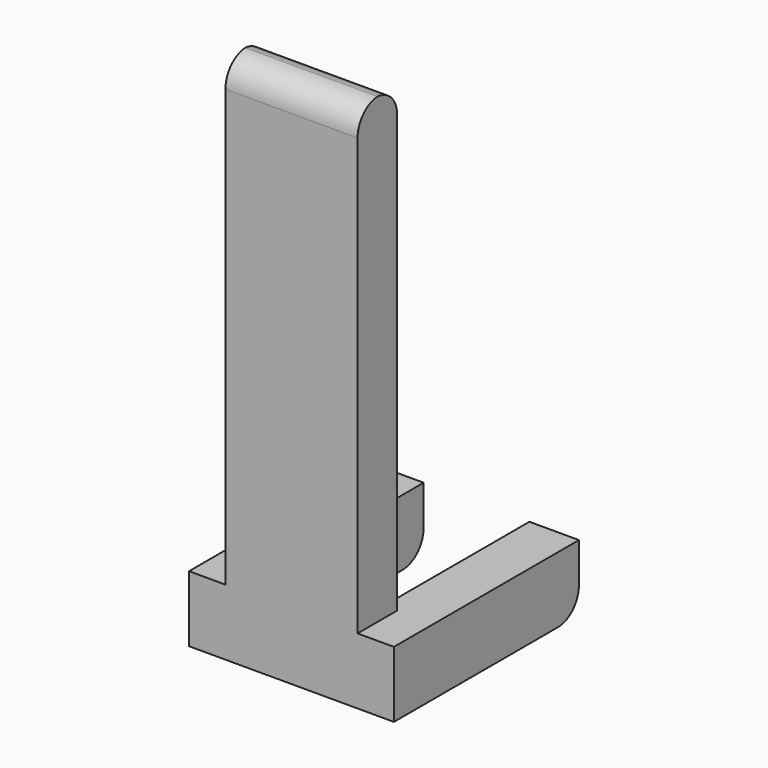
from build123d import *

# Parameters (mm, degrees)
F1_DEPTH    = 12.7
F3_DEPTH    = 88.9
F4_T1_DEPTH = 50.8
F5_R        = 5.08


# Not quite as in the source:
# - a fillet or chamfer that OpenCascade refuses, or shapes differently, is made with other operations: its cross-section is extruded or revolved along the edge and cut away or added
# - a feature names something its author has since deleted; it is built from what else it names


with BuildPart() as f1:
    # F0 (on Top) → F1 (new body)
    with BuildSketch(Plane.XY):
        Polygon((10.16, 12.7), (10.16, -12.7), (-10.16, -12.7), (-10.16, 12.7), (-10.16, 22.225), (-19.685, 22.225), (-19.685, -22.225), (19.685, -22.225), (19.685, 22.225), (10.16, 22.225), align=None)
    extrude(amount=-F1_DEPTH)

    # F2 (on face) → F3 (join)
    with BuildSketch(Plane.XY):
        Polygon((-12.7, -12.7), (-12.7, -22.225), (12.7, -22.225), (12.7, -12.7), (10.16, -12.7), (-10.16, -12.7), align=None)
    extrude(amount=F3_DEPTH)

    # F4: fillet of radius 5.08 on 2 edges, made by hand

    # F4_s2 → F4_t1 (cut)
    with BuildSketch(Plane.YZ.offset(-25.4)):
        with BuildLine():
            ThreePointArc((-12.7, 83.82), (-14.1878975516, 87.4121024484), (-17.78, 88.9))
            Line((-17.78, 88.9), (-12.7, 88.9))
            Line((-12.7, 88.9), (-12.7, 83.82))
        make_face()
        with BuildLine():
            ThreePointArc((-22.225, 83.82), (-20.7371024484, 87.4121024484), (-17.145, 88.9))
            Line((-17.145, 88.9), (-22.225, 88.9))
            Line((-22.225, 88.9), (-22.225, 83.82))
        make_face()
    extrude(amount=F4_T1_DEPTH, mode=Mode.SUBTRACT)

    # F5
    f5_edges = [f1.edges().sort_by_distance(p)[0] for p in [
        (14.9225, 22.225, -12.7),
        (-14.9225, 22.225, -12.7),
    ]]
    fillet(f5_edges, radius=F5_R)


solid = f1.part
